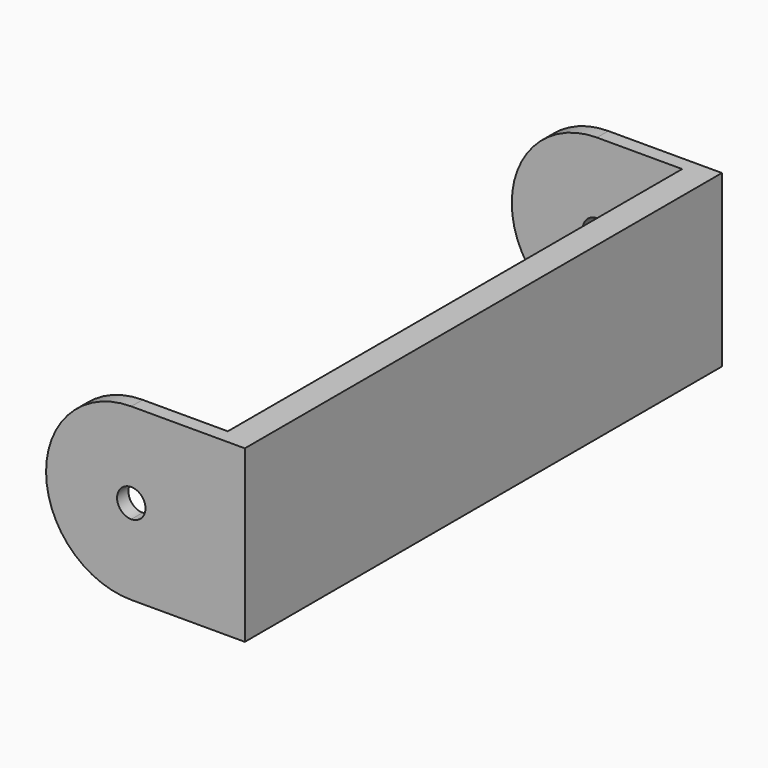
from build123d import *

# Parameters (mm, degrees)
F1_DEPTH = 5.25
F3_DEPTH = 5


# Not quite as in the source:
# - a feature names something its author has since deleted; it is built from what else it names


with BuildPart() as f1:
    # F0 (on Front) → F1 (new body, symmetric)
    with BuildSketch(Plane.XZ):
        with BuildLine():
            Line((-1, 0.25), (-1, 1.5))
            ThreePointArc((-1, 1.5), (-2.5, 0), (-1, -1.5))
            Line((-1, -1.5), (-1, -0.25))
            ThreePointArc((-1, -0.25), (-1.25, 0), (-1, 0.25))
        make_face()
        with BuildLine():
            ThreePointArc((0.5, 0), (0.0606601718, 1.0606601718), (-1, 1.5))
            Line((-1, 1.5), (-1, 0.25))
            ThreePointArc((-1, 0.25), (-0.8232233047, 0.1767766953), (-0.75, 0))
            ThreePointArc((-0.75, 0), (-0.8232233047, -0.1767766953), (-1, -0.25))
            Line((-1, -0.25), (-1, -1.5))
            ThreePointArc((-1, -1.5), (0.0606601718, -1.0606601718), (0.5, 0))
        make_face()
        with BuildLine():
            Line((1, 1.5), (-1, 1.5))
            ThreePointArc((-1, 1.5), (0.0606601718, 1.0606601718), (0.5, 0))
            ThreePointArc((0.5, 0), (0.0606601718, -1.0606601718), (-1, -1.5))
            Line((-1, -1.5), (1, -1.5))
            Line((1, -1.5), (1, 1.5))
        make_face()
    extrude(amount=F1_DEPTH, both=True)

    # F2 (on face) → F3 (cut, symmetric)
    with BuildSketch(Plane.XY.offset(1.5)):
        Polygon((-1, -4.9999998882), (0.5, -4.9999998882), (0.5, 4.9999998882), (-1, 4.9999998882), (-6.6263522021, 4.9999998882), (-6.6263522021, -4.9999998882), align=None)
    extrude(amount=F3_DEPTH, both=True, mode=Mode.SUBTRACT)


solid = f1.part
